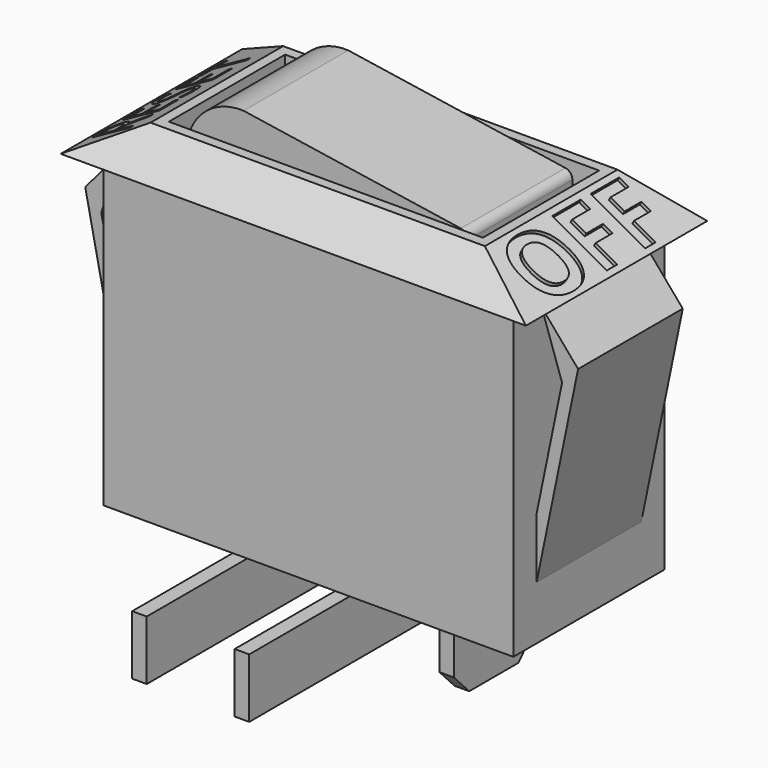
from build123d import *

# Parameters (mm, degrees)
F0_W          = 28.2
F0_H          = 21.2
F1_DEPTH      = 6.5
F2_W          = 32
F2_H          = 15.6
F2_W_2        = 28.2
F2_H_2        = 13
F3_DEPTH      = 2.5
F4_W          = 21.6
F4_H          = 10
F5_DEPTH      = 2
F8_DEPTH      = 9
F10_DEPTH     = 32.001
F13_DEPTH     = 15.601
F16_DEPTH     = 9
F17_W         = 1
F17_H         = 9
F18_DEPTH     = 6
F20_DEPTH     = 24.502829195
F22_DEPTH     = 1
F24_DEPTH     = 1
F25_TEXT_SIZE = 6.0088391948
F26_DEPTH     = 0.25
F27_TEXT_SIZE = 4.1551696153
F28_DEPTH     = 0.25


# Not quite as in the source:
# - Text() gives the source's letters only with a copy of the font that has no kerning and outlines rounded to 1/6400 em; it was checked with that copy


with BuildPart() as f1:
    # F0 (on Front) → F1 (new body, symmetric)
    with BuildSketch(Plane.XZ):
        Rectangle(F0_W, F0_H)
    extrude(amount=F1_DEPTH, both=True)

    # F2 (on face) → F3 (join)
    with BuildSketch(Plane.XY.offset(10.6)):
        Rectangle(F2_W, F2_H)
        Rectangle(F2_W_2, F2_H_2, mode=Mode.SUBTRACT)
        Rectangle(F2_W_2, F2_H_2)
    extrude(amount=F3_DEPTH)

    # F4 (on face) → F5 (cut)
    with BuildSketch(Plane.XY.offset(13.1)):
        Rectangle(F4_W, F4_H)
    extrude(amount=-F5_DEPTH, mode=Mode.SUBTRACT)

    # F7 (on offset) → F8 (join)
    with BuildSketch(Plane.XZ.offset(-4.5)):
        with BuildLine():
            ThreePointArc((-6.0605062172, 15.1), (-8.922810589, 13.9815539032), (-9.9906846881, 11.1))
            Line((-9.9906846881, 11.1), (9.3627031893, 11.1))
            Line((9.3627031893, 11.1), (9.3627031893, 12.2720245913))
            ThreePointArc((9.3627031893, 12.2720245913), (9.2251616944, 12.6429651394), (8.8790348887, 12.8345657327))
            Line((8.8790348887, 12.8345657327), (-6.0605062172, 15.1))
        make_face()
    extrude(amount=F8_DEPTH)

    # F9 (on face) → F10 (cut, through all)
    with BuildSketch(Plane.YZ.offset(16)):
        Polygon((-5.7, 13.1), (-7.8, 13.1), (-7.8, 10.6), align=None)
        Polygon((5.7, 13.1), (7.8, 10.6), (7.8, 13.1), align=None)
    extrude(amount=-F10_DEPTH, mode=Mode.SUBTRACT)

    # F12 (on offset) → F13 (cut, through all)
    with BuildSketch(Plane.XZ.offset(7.8)):
        Polygon((-11.5, 13.1), (-16, 13.1), (-16, 10.6), align=None)
        Polygon((16, 13.1), (11.5, 13.1), (16, 10.6), align=None)
    extrude(amount=-F13_DEPTH, mode=Mode.SUBTRACT)

    # F15 (on offset) → F16 (join)
    with BuildSketch(Plane.XZ.offset(4.5)):
        Polygon((-16.951829195, 6.9426484406), (-14.1, -6.8924776278), (-14.1, -2.7307082927), (-15.8492531627, 5.7554724626), (-14.4516946748, 9.8675200716), align=None)
        Polygon((14.1, -2.7307082927), (14.1, -6.8924776278), (16.951829195, 6.9426484406), (14.4516946748, 9.8675200716), (15.8492531627, 5.7554724626), align=None)
    extrude(amount=-F16_DEPTH)

    # F17 (on face) → F18 (join)
    with BuildSketch(Plane(origin=(0, 0, -10.6), x_dir=(1, 0, 0), z_dir=(0, 0, -1))):
        with Locations((-7.05, 0)):
            Rectangle(F17_W, F17_H)
        Rectangle(F17_W, F17_H)
        with Locations((7.05, 0)):
            Rectangle(F17_W, F17_H)
    extrude(amount=F18_DEPTH)

    # F19 (on face) → F20 (cut, through all)
    with BuildSketch(Plane.YZ.offset(7.55)):
        with BuildLine():
            Line((-4.5, -11.0151162371), (-4.5, -16.6))
            Line((-4.5, -16.6), (-2.1087208297, -16.6))
            Line((-2.1087208297, -16.6), (-3.4232513599, -15.2330768291))
            Line((-3.4232513599, -15.2330768291), (-3.4232513599, -11.9679604653))
            ThreePointArc((-3.4232513599, -11.9679604653), (-3.6851471488, -11.1791075534), (-4.5, -11.0151162371))
        make_face()
        with BuildLine():
            Line((3.4232513599, -15.2330768291), (2.1087208297, -16.6))
            Line((2.1087208297, -16.6), (4.5, -16.6))
            Line((4.5, -16.6), (4.5, -11.0151162371))
            ThreePointArc((4.5, -11.0151162371), (3.6851471488, -11.1791075534), (3.4232513599, -11.9679604653))
            Line((3.4232513599, -11.9679604653), (3.4232513599, -15.2330768291))
        make_face()
    extrude(amount=-F20_DEPTH, mode=Mode.SUBTRACT)

    # F21 (on face) → F22 (join)
    with BuildSketch(Plane.YZ.offset(0.5)):
        Polygon((-12.2133931145, -16.6426077485), (-4.872766789, -16.6426077485), (4.872766789, -16.6426077485), (4.872766789, -12.5524643809), (-4.872766789, -12.5524643809), (-12.2133931145, -12.5524643809), align=None)
    extrude(amount=-F22_DEPTH)

    # F23 (on face) → F24 (join)
    with BuildSketch(Plane(origin=(-7.55, 0, 0), x_dir=(0, -1, 0), z_dir=(-1, 0, 0))):
        Polygon((-3.4232513599, -12.5524643809), (-4.872766789, -12.5524643809), (-4.872766789, -16.6426077485), (12.2133931145, -16.6426077485), (12.2133931145, -12.5524643809), (3.4232513599, -12.5524643809), (3.4232513599, -15.2330768291), (2.1087208297, -16.6), (-2.1087208297, -16.6), (-3.4232513599, -15.2330768291), align=None)
    extrude(amount=-F24_DEPTH)

    # F25 (on face) → F26 (cut)
    with BuildSketch(Plane(origin=(8.2735849057, 0, 14.8924528302), x_dir=(0.8741572761, 0, -0.4856429312), z_dir=(0.4856429312, 0, 0.8741572761))):
        with Locations(Location((8.4172507833, -5.7000000961), (0, 0, 90))):
            Text('OFF', F25_TEXT_SIZE, font='Open Sans', font_style=FontStyle.BOLD, text_align=(TextAlign.LEFT, TextAlign.BOTTOM))
    extrude(amount=-F26_DEPTH, mode=Mode.SUBTRACT)

    # F27 (on face) → F28 (cut)
    with BuildSketch(Plane(origin=(-8.2735849057, 0, 14.8924528302), x_dir=(0.8741572761, 0, 0.4856429312), z_dir=(-0.4856429312, 0, 0.8741572761))):
        with Locations(Location((-5.4169789243, -6.0103889555), (0, 0, 90))):
            Text('RESET', F27_TEXT_SIZE, font='Open Sans', text_align=(TextAlign.LEFT, TextAlign.BOTTOM))
    extrude(amount=-F28_DEPTH, mode=Mode.SUBTRACT)


solid = f1.part
